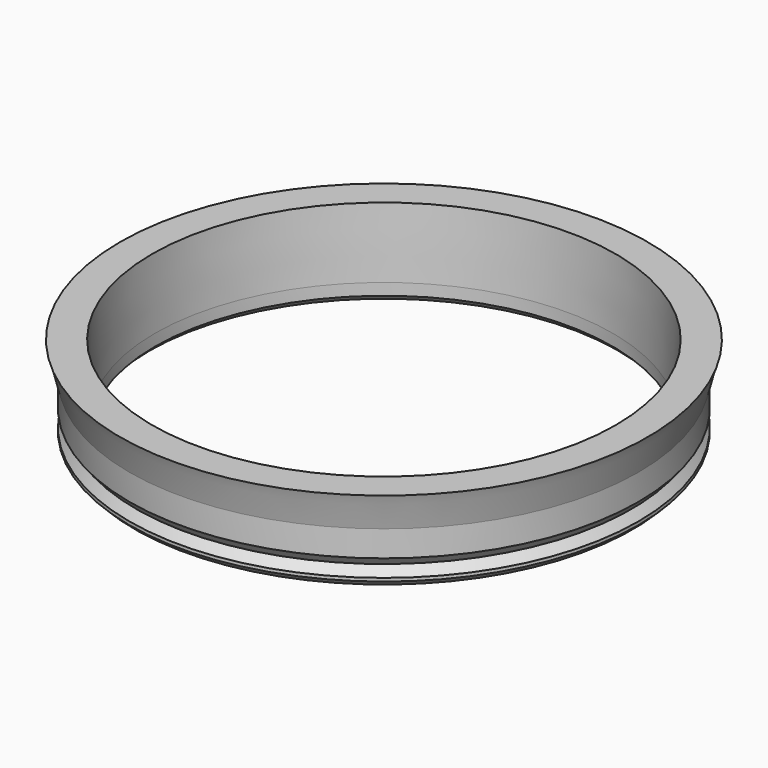
from build123d import *

# Parameters (mm, degrees)
F2_SIZE = 1.6


# Not quite as in the source:
# - a feature names something its author has since deleted; it is built from what else it names


with BuildPart() as f1:
    # F0 (on Front) → F1 (revolve)
    with BuildSketch(Plane.XZ):
        with BuildLine():
            Line((-74, 2.5490417611), (-74, 0))
            Line((-74, 0), (-67, 0))
            Line((-67, 0), (-66.5397158787, 0))
            Line((-66.5397158787, 0), (-66.5397158787, 5))
            Line((-66.5397158787, 5), (-67.375109026, 25.0225278729))
            Line((-67.375109026, 25.0225278729), (-76.7276180841, 25.0225278729))
            add(Edge.make_bspline(
                [(-74, 15.0980835222), (-74.5290090501, 18.1522390297), (-75.5065289435, 21.7678404443), (-76.7276180841, 25.0225278729)],
                knots=[0, 0, 0, 0, 0.3708554891, 0.3708554891, 0.3708554891, 0.3708554891], degree=3))
            Line((-74, 15.0980835222), (-74, 7.5490417611))
            Line((-74, 7.5490417611), (-72, 5.0490417611))
            Line((-72, 5.0490417611), (-74, 2.5490417611))
        make_face()
    revolve(axis=Axis((0, 0, 30.7617206126), (0, 0, 1)))

    # F2
    f2_edges = [f1.edges().sort_by_distance(p)[0] for p in [
        (74, 0, 0),
        (66.539716, 0, 0),
    ]]
    chamfer(f2_edges, length=F2_SIZE)


solid = f1.part
